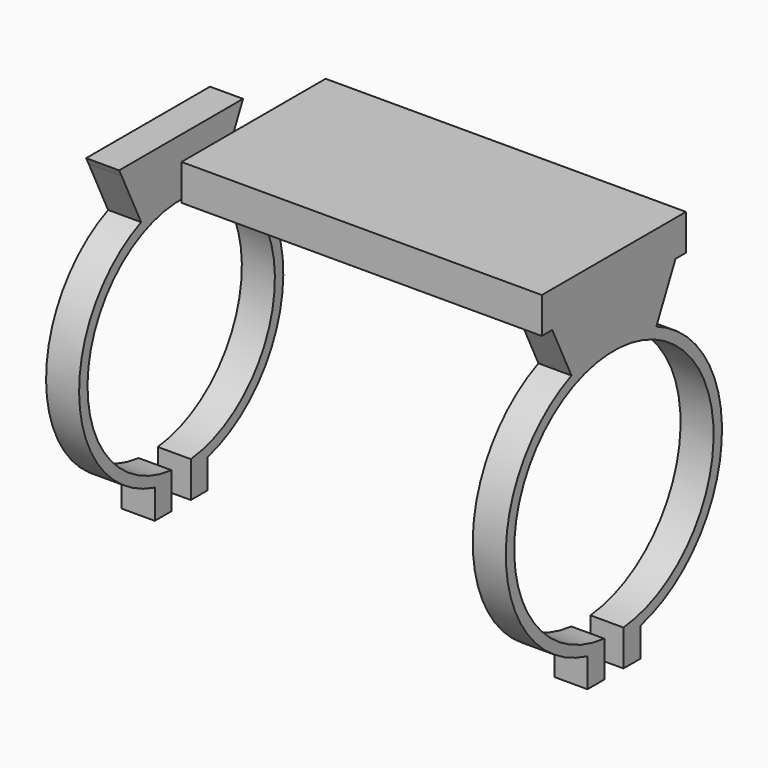
from build123d import *

# Parameters (mm, degrees)
F2_W     = 120
F2_H     = 60
F3_DEPTH = 12
F5_DEPTH = 11
F7_DEPTH = 5.5


# Not quite as in the source:
# - a feature names something its author has since deleted; it is built from what else it names
# - the program builds the solid bodies; features that only make, move or delete a surface that nothing else refers to are left out


with BuildPart() as f3:
    # F2 (on Top) → F3 (new body)
    with BuildSketch(Plane.XY):
        with Locations((-7, 0)):
            Rectangle(F2_W, F2_H)
    extrude(amount=-F3_DEPTH)

    # F4 (on face) → F5 (join)
    with BuildSketch(Plane.YZ.offset(53)):
        with BuildLine():
            ThreePointArc((-17.6681073643, -28.6135531585), (0, -25), (17.6681073643, -28.6135531585))
            Line((17.6681073643, -28.6135531585), (25.6533360622, -12))
            Line((25.6533360622, -12), (-25.6533360622, -12))
            Line((-25.6533360622, -12), (-17.6681073643, -28.6135531585))
        make_face()
        Polygon((-25.6533360622, -12), (25.6533360622, -12), (25.762218982, -11.7734652013), (0, -11.7734652013), (-25.762218982, -11.7734652013), align=None)
        with BuildLine():
            ThreePointArc((-4, -111.3067791046), (0, -28.5), (4, -111.3067791046))
            Line((4, -111.3067791046), (11, -111.3067791046))
            Line((11, -111.3067791046), (11, -113.6348484585))
            ThreePointArc((11, -113.6348484585), (44.8622364421, -73.5184856705), (17.6681073643, -28.6135531585))
            ThreePointArc((17.6681073643, -28.6135531585), (0, -25), (-17.6681073643, -28.6135531585))
            ThreePointArc((-17.6681073643, -28.6135531585), (-44.8622364421, -73.5184856705), (-11, -113.6348484585))
            Line((-11, -113.6348484585), (-11, -111.3067791046))
            Line((-11, -111.3067791046), (-4, -111.3067791046))
        make_face()
        with BuildLine():
            Line((-4, -123.3067791046), (-4, -114.821869662))
            ThreePointArc((-4, -114.821869662), (-7.5234470048, -114.3666287334), (-11, -113.6348484585))
            Line((-11, -113.6348484585), (-11, -123.3067791046))
            Line((-11, -123.3067791046), (-4, -123.3067791046))
        make_face()
        with BuildLine():
            ThreePointArc((11, -113.6348484585), (7.5234470048, -114.3666287334), (4, -114.821869662))
            Line((4, -114.821869662), (4, -123.3067791046))
            Line((4, -123.3067791046), (11, -123.3067791046))
            Line((11, -123.3067791046), (11, -113.6348484585))
        make_face()
        with BuildLine():
            Line((11, -111.3067791046), (4, -111.3067791046))
            Line((4, -111.3067791046), (4, -114.821869662))
            ThreePointArc((4, -114.821869662), (7.5234470048, -114.3666287334), (11, -113.6348484585))
            Line((11, -113.6348484585), (11, -111.3067791046))
        make_face()
        with BuildLine():
            Line((-4, -114.821869662), (-4, -111.3067791046))
            Line((-4, -111.3067791046), (-11, -111.3067791046))
            Line((-11, -111.3067791046), (-11, -113.6348484585))
            ThreePointArc((-11, -113.6348484585), (-7.5234470048, -114.3666287334), (-4, -114.821869662))
        make_face()
    extrude(amount=-F5_DEPTH)


with BuildPart() as f7:
    # F6 (on face) → F7 (new body, symmetric)
    with BuildSketch(Plane(origin=(-67, 0, 0), x_dir=(0, -1, 0), z_dir=(-1, 0, 0))):
        with BuildLine():
            ThreePointArc((-4, -108.7943294825), (0, -31), (4, -108.7943294825))
            Line((4, -108.7943294825), (11, -108.7943294825))
            Line((11, -108.7943294825), (11, -111.0517965502))
            ThreePointArc((11, -111.0517965502), (42.393406197, -73.0081740329), (16.686545844, -30.9128002052))
            ThreePointArc((16.686545844, -30.9128002052), (0, -27.5), (-16.686545844, -30.9128002052))
            ThreePointArc((-16.686545844, -30.9128002052), (-42.393406197, -73.0081740329), (-11, -111.0517965502))
            Line((-11, -111.0517965502), (-11, -108.7943294825))
            Line((-11, -108.7943294825), (-4, -108.7943294825))
        make_face()
        with BuildLine():
            Line((-4, -112.3113459961), (-4, -108.7943294825))
            Line((-4, -108.7943294825), (-11, -108.7943294825))
            Line((-11, -108.7943294825), (-11, -111.0517965502))
            ThreePointArc((-11, -111.0517965502), (-7.526394635, -111.8282605878), (-4, -112.3113459961))
        make_face()
        with BuildLine():
            Line((-4, -120.7943294825), (-4, -112.3113459961))
            ThreePointArc((-4, -112.3113459961), (-7.526394635, -111.8282605878), (-11, -111.0517965502))
            Line((-11, -111.0517965502), (-11, -118.8568006338))
            Line((-11, -118.8568006338), (-11, -120.7943294825))
            Line((-11, -120.7943294825), (-4, -120.7943294825))
        make_face()
        with BuildLine():
            Line((11, -108.7943294825), (4, -108.7943294825))
            Line((4, -108.7943294825), (4, -112.3113459961))
            ThreePointArc((4, -112.3113459961), (7.526394635, -111.8282605878), (11, -111.0517965502))
            Line((11, -111.0517965502), (11, -108.7943294825))
        make_face()
        with BuildLine():
            ThreePointArc((11, -111.0517965502), (7.526394635, -111.8282605878), (4, -112.3113459961))
            Line((4, -112.3113459961), (4, -120.7943294825))
            Line((4, -120.7943294825), (11, -120.7943294825))
            Line((11, -120.7943294825), (11, -111.0517965502))
        make_face()
        with BuildLine():
            ThreePointArc((-16.686545844, -30.9128002052), (0, -27.5), (16.686545844, -30.9128002052))
            Line((16.686545844, -30.9128002052), (24.7806574617, -14.072712248))
            Line((24.7806574617, -14.072712248), (25.8327852935, -12))
            Line((25.8327852935, -12), (-25.743663311, -12))
            Line((-25.743663311, -12), (-24.7806574617, -14.072712248))
            Line((-24.7806574617, -14.072712248), (-16.686545844, -30.9128002052))
        make_face()
    extrude(amount=F7_DEPTH, both=True)


with BuildPart() as f7_1:
    # F8: moved
    add(f7.part.moved(Location((-29.6, 0, 0))))


solid = Compound([f3.part, f7_1.part])
